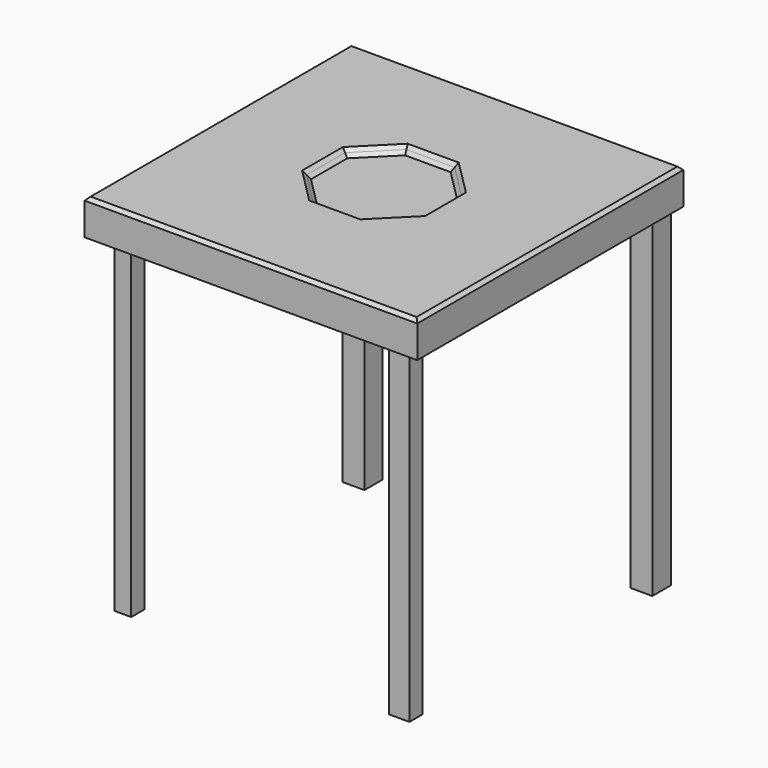
from build123d import *

# Parameters (mm, degrees)
F0_W      = 1000
F0_H      = 1000
F1_DEPTH  = 100
F3_DEPTH  = 20
F4_SIZE   = 9.99999
F5_W      = 50
F5_H      = 50
F6_DEPTH  = 1000
F7_W      = 61.6666623382
F7_H      = 50
F8_DEPTH  = 1000
F9_W      = 1000
F9_H      = 1000
F9_W_2    = 50
F9_H_2    = 50
F9_W_3    = 61.6666623382
F10_W     = 57.3770701885
F10_H     = 57.3770701885
F10_W_2   = 65.0272965431
F10_H_2   = 76.5027403831
F11_DEPTH = 7
F12_W     = 66.2613213062
F12_H     = 68.3319568634
F13_DEPTH = 1000
F14_W     = 65.0273263454
F14_H     = 70.7650482655
F15_DEPTH = 1000


# Not quite as in the source:
# - a fillet or chamfer is up to 0.001 mm smaller than in the source, because OpenCascade refuses the exact size


with BuildPart() as f1:
    # F0 (on Top) → F1 (new body)
    with BuildSketch(Plane.XY):
        Rectangle(F0_W, F0_H)
    extrude(amount=F1_DEPTH)

    # F2 (on face) → F3 (cut)
    with BuildSketch(Plane.XY.offset(100)):
        Polygon((72.4873734153, -175), (175, -72.4873734153), (175, 72.4873734153), (72.4873734153, 175), (-72.4873734153, 175), (-175, 72.4873734153), (-175, -72.4873734153), (-72.4873734153, -175), align=None)
    extrude(amount=-F3_DEPTH, mode=Mode.SUBTRACT)

    # F4 (size 10 in the source; OpenCascade refuses exactly that, so slightly less here)
    f4_edges = [f1.edges().sort_by_distance(p)[0] for p in [
        (123.743687, -123.743687, 80),
        (175, 0, 80),
        (123.743687, 123.743687, 80),
        (0, 175, 80),
        (-123.743687, 123.743687, 80),
        (-175, 0, 80),
        (-123.743687, -123.743687, 80),
        (0, -175, 80),
        (0, -500, 100),
        (-500, 0, 100),
        (500, 0, 100),
        (0, 500, 100),
        (123.743687, -123.743687, 100),
        (175, 0, 100),
        (123.743687, 123.743687, 100),
        (0, 175, 100),
        (-123.743687, 123.743687, 100),
        (-175, 0, 100),
        (-123.743687, -123.743687, 100),
        (0, -175, 100),
    ]]
    chamfer(f4_edges, length=F4_SIZE)

    # F5 (on face) → F6 (join)
    with BuildSketch(Plane(origin=(0, 0, 0), x_dir=(1, 0, 0), z_dir=(0, 0, -1))):
        with Locations((-425, 425)):
            Rectangle(F5_W, F5_H)
    extrude(amount=F6_DEPTH)

    # F7 (on face) → F8 (join)
    with BuildSketch(Plane(origin=(0, 0, 0), x_dir=(1, 0, 0), z_dir=(0, 0, -1))):
        with Locations((412.1584743261, 433.19670856)):
            Rectangle(F7_W, F7_H)
    extrude(amount=F8_DEPTH)

    # F9 (on face) + F10 (on face) → F11 (join)
    with BuildSketch(Plane(origin=(0, 0, 0), x_dir=(1, 0, 0), z_dir=(0, 0, -1))):
        Rectangle(F9_W, F9_H)
        with Locations((-425, 425)):
            Rectangle(F9_W_2, F9_H_2, mode=Mode.SUBTRACT)
        with Locations((412.1584743261, 433.19670856)):
            Rectangle(F9_W_3, F9_H_2, mode=Mode.SUBTRACT)
    with BuildSketch(Plane(origin=(0, 0, 0), x_dir=(1, 0, 0), z_dir=(0, 0, -1))):
        with Locations((-409.2896133661, -459.9726945162)):
            Rectangle(F10_W, F10_H)
        with Locations((434.1530203819, -438.9344155788)):
            Rectangle(F10_W_2, F10_H_2)
    extrude(amount=F11_DEPTH)

    # F12 (on face) → F13 (join)
    with BuildSketch(Plane(origin=(0, 0, -7), x_dir=(1, 0, 0), z_dir=(0, 0, -1))):
        with Locations((-417.2714799643, -440.7140314579)):
            Rectangle(F12_W, F12_H)
    extrude(amount=F13_DEPTH)

    # F14 (on face) → F15 (join)
    with BuildSketch(Plane(origin=(0, 0, -7), x_dir=(1, 0, 0), z_dir=(0, 0, -1))):
        with Locations((447.5409835577, -443.7158554792)):
            Rectangle(F14_W, F14_H)
    extrude(amount=F15_DEPTH)


solid = f1.part
